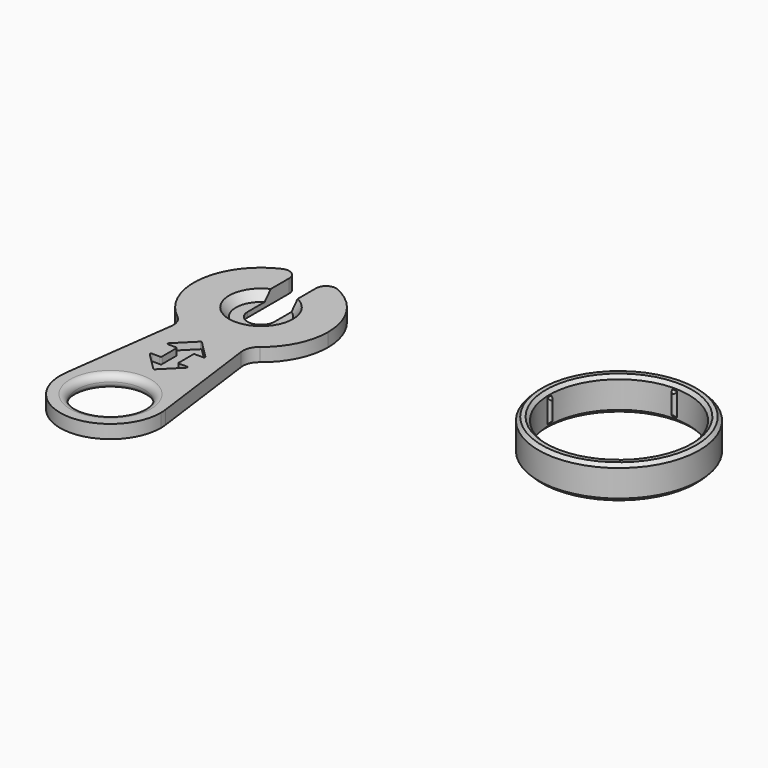
from build123d import *

# Parameters (mm, degrees)
F1_R         = 24
F1_R_2       = 20.75
F2_DEPTH     = 10
F3_SIZE      = 1
F5_R         = 0.7
F6_DEPTH     = 2.5
F7_T4_ANGLE  = 18.0680133359
F7_S5_R      = 0.7
F7_T6_DEPTH  = 5
F7_T10_ANGLE = 18.0680133359
F7_S11_R     = 0.7
F7_T12_DEPTH = 5
F7_T16_ANGLE = 9.0340027216
F7_S17_R     = 0.7
F7_T18_DEPTH = 3
F7_T22_ANGLE = 9.0340027216
F7_S23_R     = 0.7
F7_T24_DEPTH = 3
F7_T28_ANGLE = 18.0680133359
F7_S29_R     = 0.7
F7_T30_DEPTH = 5
F7_T34_ANGLE = 18.0680133359
F7_S35_R     = 0.7
F7_T36_DEPTH = 5
F7_T40_ANGLE = 9.0340027216
F7_S41_R     = 0.7
F7_T42_DEPTH = 3
F7_T46_ANGLE = 9.0340027216
F7_S47_R     = 0.7
F7_T48_DEPTH = 3
F7_T52_ANGLE = 18.0680133359
F7_S53_R     = 0.7
F7_T54_DEPTH = 5
F7_T58_ANGLE = 18.0680133359
F7_S59_R     = 0.7
F7_T60_DEPTH = 5
F8_R         = 4
F8_R_2       = 10
F9_DEPTH     = 4
F10_R        = 9.5
F10_R_2      = 4
F11_DEPTH    = 2.5
F14_DEPTH    = 4.001
F15_R        = 3
F16_R        = 5
F17_R        = 1.99999
F19_DEPTH    = 2
F20_R        = 0.3


# Not quite as in the source:
# - a fillet or chamfer that OpenCascade refuses, or shapes differently, is made with other operations: its cross-section is extruded or revolved along the edge and cut away or added
# - a fillet or chamfer is up to 0.001 mm smaller than in the source, because OpenCascade refuses the exact size
# - a feature names something its author has since deleted; it is built from what else it names


with BuildPart() as f2:
    # F1 (on Top) → F2 (new body)
    with BuildSketch(Plane.XY):
        Circle(F1_R)
        Circle(F1_R_2, mode=Mode.SUBTRACT)
    extrude(amount=F2_DEPTH)

    # F3
    f3_edges = [f2.edges().sort_by_distance(p)[0] for p in [
        (-20.75, 0, 10),
        (-20.75, 0, 0),
        (-24, 0, 10),
        (-24, 0, 0),
    ]]
    chamfer(f3_edges, length=F3_SIZE)

    # F5 (on offset) → F6 (join, symmetric)
    with BuildSketch(Plane.XY.offset(5)):
        with Locations((-20.75, 0)):
            Circle(F5_R)
        with Locations((0, -20.75)):
            Circle(F5_R)
        with Locations((20.75, 0)):
            Circle(F5_R)
        with Locations((0, 20.75)):
            Circle(F5_R)
    extrude(amount=F6_DEPTH, both=True)

    # F7: chamfer of 1 on 10 edges, made by hand


with BuildPart() as f7_tool2:
    # F7_s3 → F7_t4 (revolve)
    with BuildSketch(Plane(origin=(0, 0, 0), x_dir=(0, 0, 1), z_dir=(-0.9875953183, -0.1570206585, 0))):
        Polygon((8.5, 20.75), (7.5, 19.75), (7.5, 20.75), align=None)
    revolve(axis=Axis((0, 0, 7.5), (0, 0, -1)), revolution_arc=F7_T4_ANGLE)

    # F7_s5 → F7_t6 (intersect, symmetric)
    with BuildSketch(Plane.XY.offset(8)):
        with Locations((0, 20.75)):
            Circle(F7_S5_R)
    extrude(amount=F7_T6_DEPTH, both=True, mode=Mode.INTERSECT)


with BuildPart() as f2_1:
    add(f2.part)

    # F7_t1: union F7_tool2
    add(f7_tool2.part)


with BuildPart() as f7_tool8:
    # F7_s9 → F7_t10 (revolve)
    with BuildSketch(Plane(origin=(0, 0, 0), x_dir=(0, 0, 1), z_dir=(0.1570206585, -0.9875953183, 0))):
        Polygon((8.5, 20.75), (7.5, 19.75), (7.5, 20.75), align=None)
    revolve(axis=Axis((0, 0, 7.5), (0, 0, -1)), revolution_arc=F7_T10_ANGLE)

    # F7_s11 → F7_t12 (intersect, symmetric)
    with BuildSketch(Plane.XY.offset(8)):
        with Locations((-20.75, 0)):
            Circle(F7_S11_R)
    extrude(amount=F7_T12_DEPTH, both=True, mode=Mode.INTERSECT)


with BuildPart() as f2_2:
    add(f2_1.part)

    # F7_t7: union F7_tool8
    add(f7_tool8.part)


with BuildPart() as f7_tool14:
    # F7_s15 → F7_t16 (revolve)
    with BuildSketch(Plane.XZ):
        Polygon((20.75, 8.5), (19.75, 7.5), (20.75, 7.5), align=None)
    revolve(axis=Axis((0, 0, 7.5), (0, 0, -1)), revolution_arc=F7_T16_ANGLE)

    # F7_s17 → F7_t18 (intersect, symmetric)
    with BuildSketch(Plane.XY.offset(8)):
        with Locations((20.75, 0)):
            Circle(F7_S17_R)
    extrude(amount=F7_T18_DEPTH, both=True, mode=Mode.INTERSECT)


with BuildPart() as f2_3:
    add(f2_2.part)

    # F7_t13: union F7_tool14
    add(f7_tool14.part)


with BuildPart() as f7_tool20:
    # F7_s21 → F7_t22 (revolve)
    with BuildSketch(Plane(origin=(0, 0, 0), x_dir=(0, 0, 1), z_dir=(-0.1570205904, 0.9875953292, 0))):
        Polygon((8.5, 20.75), (7.5, 19.75), (7.5, 20.75), align=None)
    revolve(axis=Axis((0, 0, 7.5), (0, 0, -1)), revolution_arc=F7_T22_ANGLE)

    # F7_s23 → F7_t24 (intersect, symmetric)
    with BuildSketch(Plane.XY.offset(8)):
        with Locations((20.75, 0)):
            Circle(F7_S23_R)
    extrude(amount=F7_T24_DEPTH, both=True, mode=Mode.INTERSECT)


with BuildPart() as f2_4:
    add(f2_3.part)

    # F7_t19: union F7_tool20
    add(f7_tool20.part)


with BuildPart() as f7_tool26:
    # F7_s27 → F7_t28 (revolve)
    with BuildSketch(Plane(origin=(0, 0, 0), x_dir=(0, 0, 1), z_dir=(0.9875953183, 0.1570206585, 0))):
        Polygon((8.5, 20.75), (7.5, 19.75), (7.5, 20.75), align=None)
    revolve(axis=Axis((0, 0, 7.5), (0, 0, -1)), revolution_arc=F7_T28_ANGLE)

    # F7_s29 → F7_t30 (intersect, symmetric)
    with BuildSketch(Plane.XY.offset(8)):
        with Locations((0, -20.75)):
            Circle(F7_S29_R)
    extrude(amount=F7_T30_DEPTH, both=True, mode=Mode.INTERSECT)


with BuildPart() as f2_5:
    add(f2_4.part)

    # F7_t25: union F7_tool26
    add(f7_tool26.part)


with BuildPart() as f7_tool32:
    # F7_s33 → F7_t34 (revolve)
    with BuildSketch(Plane(origin=(0, 0, 0), x_dir=(0, 0, 1), z_dir=(-0.9875953183, -0.1570206585, 0))):
        Polygon((1.5, 20.75), (2.5, 19.75), (2.5, 20.75), align=None)
    revolve(axis=Axis((0, 0, 2.5), (0, 0, -1)), revolution_arc=F7_T34_ANGLE)

    # F7_s35 → F7_t36 (intersect, symmetric)
    with BuildSketch(Plane.XY.offset(2)):
        with Locations((0, 20.75)):
            Circle(F7_S35_R)
    extrude(amount=F7_T36_DEPTH, both=True, mode=Mode.INTERSECT)


with BuildPart() as f2_6:
    add(f2_5.part)

    # F7_t31: union F7_tool32
    add(f7_tool32.part)


with BuildPart() as f7_tool38:
    # F7_s39 → F7_t40 (revolve)
    with BuildSketch(Plane.XZ):
        Polygon((20.75, 1.5), (19.75, 2.5), (20.75, 2.5), align=None)
    revolve(axis=Axis((0, 0, 2.5), (0, 0, -1)), revolution_arc=F7_T40_ANGLE)

    # F7_s41 → F7_t42 (intersect, symmetric)
    with BuildSketch(Plane.XY.offset(2)):
        with Locations((20.75, 0)):
            Circle(F7_S41_R)
    extrude(amount=F7_T42_DEPTH, both=True, mode=Mode.INTERSECT)


with BuildPart() as f2_7:
    add(f2_6.part)

    # F7_t37: union F7_tool38
    add(f7_tool38.part)


with BuildPart() as f7_tool44:
    # F7_s45 → F7_t46 (revolve)
    with BuildSketch(Plane(origin=(0, 0, 0), x_dir=(0, 0, 1), z_dir=(-0.1570205904, 0.9875953292, 0))):
        Polygon((1.5, 20.75), (2.5, 19.75), (2.5, 20.75), align=None)
    revolve(axis=Axis((0, 0, 2.5), (0, 0, -1)), revolution_arc=F7_T46_ANGLE)

    # F7_s47 → F7_t48 (intersect, symmetric)
    with BuildSketch(Plane.XY.offset(2)):
        with Locations((20.75, 0)):
            Circle(F7_S47_R)
    extrude(amount=F7_T48_DEPTH, both=True, mode=Mode.INTERSECT)


with BuildPart() as f2_8:
    add(f2_7.part)

    # F7_t43: union F7_tool44
    add(f7_tool44.part)


with BuildPart() as f7_tool50:
    # F7_s51 → F7_t52 (revolve)
    with BuildSketch(Plane(origin=(0, 0, 0), x_dir=(0, 0, 1), z_dir=(0.9875953183, 0.1570206585, 0))):
        Polygon((1.5, 20.75), (2.5, 19.75), (2.5, 20.75), align=None)
    revolve(axis=Axis((0, 0, 2.5), (0, 0, -1)), revolution_arc=F7_T52_ANGLE)

    # F7_s53 → F7_t54 (intersect, symmetric)
    with BuildSketch(Plane.XY.offset(2)):
        with Locations((0, -20.75)):
            Circle(F7_S53_R)
    extrude(amount=F7_T54_DEPTH, both=True, mode=Mode.INTERSECT)


with BuildPart() as f2_9:
    add(f2_8.part)

    # F7_t49: union F7_tool50
    add(f7_tool50.part)


with BuildPart() as f7_tool56:
    # F7_s57 → F7_t58 (revolve)
    with BuildSketch(Plane(origin=(0, 0, 0), x_dir=(0, 0, 1), z_dir=(0.1570206585, -0.9875953183, 0))):
        Polygon((1.5, 20.75), (2.5, 19.75), (2.5, 20.75), align=None)
    revolve(axis=Axis((0, 0, 2.5), (0, 0, -1)), revolution_arc=F7_T58_ANGLE)

    # F7_s59 → F7_t60 (intersect, symmetric)
    with BuildSketch(Plane.XY.offset(2)):
        with Locations((-20.75, 0)):
            Circle(F7_S59_R)
    extrude(amount=F7_T60_DEPTH, both=True, mode=Mode.INTERSECT)


with BuildPart() as f2_10:
    add(f2_9.part)

    # F7_t55: union F7_tool56
    add(f7_tool56.part)


with BuildPart() as f9:
    # F8 (on Top) → F9 (new body)
    with BuildSketch(Plane.XY):
        with BuildLine():
            ThreePointArc((-96.6999239548, -17.3205080757), (-89.3794158791, -10), (-86.6999239548, 0))
            ThreePointArc((-86.6999239548, 0), (-116.6999239548, 17.3205080757), (-116.6999239548, -17.3205080757))
            ThreePointArc((-116.6999239548, -17.3205080757), (-106.6999239548, -20), (-96.6999239548, -17.3205080757))
        make_face()
        with Locations((-106.6999239548, 0)):
            Circle(F8_R, mode=Mode.SUBTRACT)
        with BuildLine():
            ThreePointArc((-96.6999239548, -17.3205080757), (-106.6999239548, -20), (-116.6999239548, -17.3205080757))
            Line((-116.6999239548, -17.3205080757), (-121.5703116276, -54.1285096235))
            ThreePointArc((-121.5703116276, -54.1285096235), (-106.6999239548, -41.0961402953), (-91.829536282, -54.1285096235))
            Line((-91.829536282, -54.1285096235), (-96.6999239548, -17.3205080757))
        make_face()
        with BuildLine():
            ThreePointArc((-91.829536282, -54.1285096235), (-106.6999239548, -41.0961402953), (-121.5703116276, -54.1285096235))
            ThreePointArc((-121.5703116276, -54.1285096235), (-107.6858714453, -71.063702139), (-91.6999239548, -56.0961402953))
            ThreePointArc((-91.6999239548, -56.0961402953), (-91.7323621111, -55.1101928048), (-91.829536282, -54.1285096235))
        make_face()
        with Locations((-106.6999239548, -56.0961402953)):
            Circle(F8_R_2, mode=Mode.SUBTRACT)
    extrude(amount=F9_DEPTH)

    # F10 (on face) → F11 (cut)
    with BuildSketch(Plane.XY.offset(4)):
        with Locations((-106.6999239548, 0)):
            Circle(F10_R)
        with Locations((-106.6999239548, 0)):
            Circle(F10_R_2, mode=Mode.SUBTRACT)
    extrude(amount=-F11_DEPTH, mode=Mode.SUBTRACT)

    # F12: chamfer of 2 x 2.5 on 1 edges, made by hand


with BuildPart() as f12_tool2:
    # F12_s3 → F12_t4 (revolve)
    with BuildSketch(Plane.XZ):
        Polygon((-97.1999239548, 4), (-99.1999239548, 1.5), (-97.1999239548, 1.5), align=None)
    revolve(axis=Axis((-106.6999239548, 0, 1.5), (0, 0, 1)))

    split(bisect_by=Plane.XY.offset(4), keep=Keep.BOTTOM)


with BuildPart() as f9_1:
    add(f9.part)

    # F12_t1: union F12_tool2
    add(f12_tool2.part)

    # F13 (on face) → F14 (cut, through all)
    with BuildSketch(Plane.XY.offset(4)):
        with BuildLine():
            ThreePointArc((-110.6999239548, 19.5959179423), (-106.6999239548, 20), (-102.6999239548, 19.5959179423))
            Line((-102.6999239548, 19.5959179423), (-102.6999239548, 21))
            Line((-102.6999239548, 21), (-110.6999239548, 21))
            Line((-110.6999239548, 21), (-110.6999239548, 19.5959179423))
        make_face()
        with BuildLine():
            ThreePointArc((-110.6999239548, 8.6168439698), (-106.6999239548, 9.5), (-102.6999239548, 8.6168439698))
            Line((-102.6999239548, 8.6168439698), (-102.6999239548, 19.5959179423))
            ThreePointArc((-102.6999239548, 19.5959179423), (-106.6999239548, 20), (-110.6999239548, 19.5959179423))
            Line((-110.6999239548, 19.5959179423), (-110.6999239548, 8.6168439698))
        make_face()
        with BuildLine():
            ThreePointArc((-110.6999239548, 0), (-106.6999239548, 4), (-102.6999239548, 0))
            Line((-102.6999239548, 0), (-102.6999239548, 8.6168439698))
            ThreePointArc((-102.6999239548, 8.6168439698), (-106.6999239548, 9.5), (-110.6999239548, 8.6168439698))
            Line((-110.6999239548, 8.6168439698), (-110.6999239548, 0))
        make_face()
    extrude(amount=-F14_DEPTH, mode=Mode.SUBTRACT)

    # F15
    f15_edges = [f9_1.edges().sort_by_distance(p)[0] for p in [
        (-110.699924, 19.595918, 2),
        (-102.699924, 19.595918, 2),
    ]]
    fillet(f15_edges, radius=F15_R)

    # F16
    f16_edges = [f9_1.edges().sort_by_distance(p)[0] for p in [
        (-96.699924, -17.320508, 2),
        (-116.699924, -17.320508, 2),
    ]]
    fillet(f16_edges, radius=F16_R)

    # F17 (radius 2 in the source; OpenCascade refuses exactly that, so slightly less here)
    f17_edges = [f9_1.edges().sort_by_distance(p)[0] for p in [
        (-116.699924, -56.09614, 4),
        (-116.699924, -56.09614, 0),
    ]]
    fillet(f17_edges, radius=F17_R)

    # F18 (on face) → F19 (cut)
    with BuildSketch(Plane.XY.offset(4)):
        Polygon((-109.1999239548, -28.0961402953), (-109.1999239548, -31.0961402953), (-109.1999239548, -34.0961402953), (-112.6999239548, -34.0961402953), (-106.6999239548, -40.0961402953), (-100.6999239548, -34.0961402953), (-104.1999239548, -34.0961402953), (-104.1999239548, -31.0961402953), (-104.1999239548, -28.0961402953), (-100.6999239548, -28.0961402953), (-106.6999239548, -22.0961402953), (-112.6999239548, -28.0961402953), align=None)
    extrude(amount=-F19_DEPTH, mode=Mode.SUBTRACT)

    # F20
    f20_edges = [f9_1.edges().sort_by_distance(p)[0] for p in [
        (-112.699924, -28.09614, 3),
        (-100.699924, -28.09614, 3),
        (-100.699924, -34.09614, 3),
        (-112.699924, -34.09614, 3),
        (-109.199924, -34.09614, 3),
        (-109.199924, -28.09614, 3),
        (-104.199924, -28.09614, 3),
        (-104.199924, -34.09614, 3),
        (-106.699924, -22.09614, 3),
        (-106.699924, -40.09614, 3),
    ]]
    fillet(f20_edges, radius=F20_R)


solid = Compound([f2_10.part, f9_1.part])
